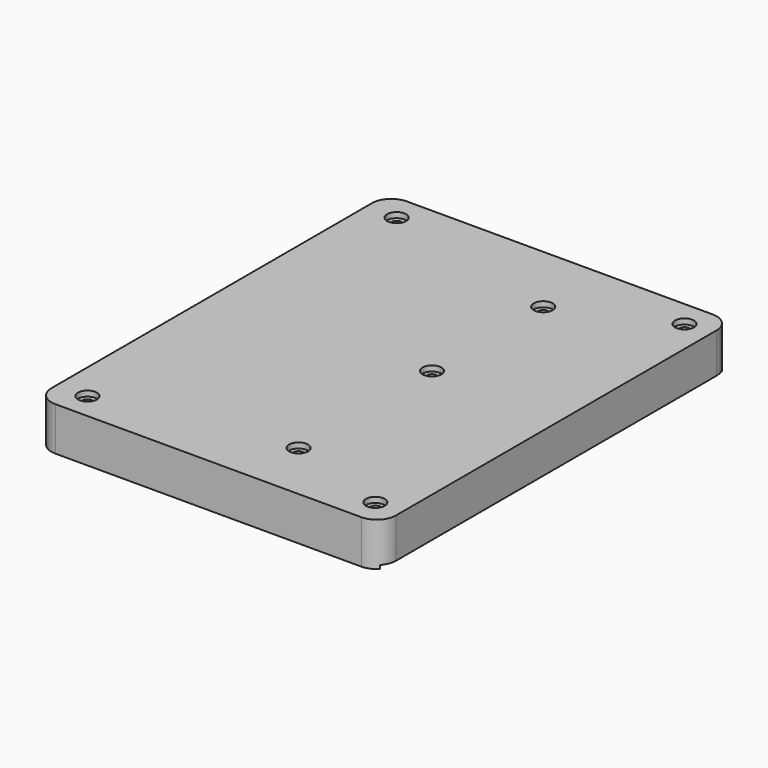
from build123d import *

# Parameters (mm, degrees)
F7_DEPTH        = 8.9
F9_DEPTH        = 0.8
F11_W           = 14.971
F11_H           = 45.903
F11_H_2         = 42.347
F13_DEPTH       = 7.1999999775
F14_DEPTH       = 5.9
F10_R           = 2.6
F16_R           = 3.5
F18_DEPTH       = 4.4
F19_SIZE        = 0.89999
F20_D           = 2.2
F20_CBORE_D     = 4.2
F20_CBORE_DEPTH = 1.2
F21_W           = 84.162
F21_H           = 95.25
F22_DEPTH       = 0.801


# Not quite as in the source:
# - a fillet or chamfer is up to 0.001 mm smaller than in the source, because OpenCascade refuses the exact size


with BuildPart() as f7:
    # F4 (on offset) → F7 (new body, through all)
    with BuildSketch(Plane.XY.offset(1.7)):
        with BuildLine():
            Line((84.612, 3), (84.612, 92.25))
            ThreePointArc((84.612, 92.25), (83.3525591591, 95.2905591591), (80.312, 96.55))
            Line((80.312, 96.55), (12.15, 96.55))
            ThreePointArc((12.15, 96.55), (9.1094408409, 95.2905591591), (7.85, 92.25))
            Line((7.85, 92.25), (7.85, 3))
            ThreePointArc((7.85, 3), (9.1094408409, -0.0405591591), (12.15, -1.3))
            Line((12.15, -1.3), (80.312, -1.3))
            ThreePointArc((80.312, -1.3), (83.3525591591, -0.0405591591), (84.612, 3))
        make_face()
    extrude(amount=F7_DEPTH)

    # F8 (on offset) → F9 (join)
    with BuildSketch(Plane.XY.offset(1.7)):
        with BuildLine():
            Line((84.612, 3), (84.612, 92.25))
            ThreePointArc((84.612, 92.25), (83.3525591591, 95.2905591591), (80.312, 96.55))
            Line((80.312, 96.55), (12.15, 96.55))
            ThreePointArc((12.15, 96.55), (9.1094408409, 95.2905591591), (7.85, 92.25))
            Line((7.85, 92.25), (7.85, 3))
            ThreePointArc((7.85, 3), (9.1094408409, -0.0405591591), (12.15, -1.3))
            Line((12.15, -1.3), (80.312, -1.3))
            ThreePointArc((80.312, -1.3), (83.3525591591, -0.0405591591), (84.612, 3))
        make_face()
        with BuildLine():
            ThreePointArc((80.312, 95.25), (82.4333203436, 94.3713203436), (83.312, 92.25))
            Line((83.312, 92.25), (83.312, 3))
            ThreePointArc((83.312, 3), (82.4333203436, 0.8786796564), (80.312, 0))
            Line((80.312, 0), (12.15, 0))
            ThreePointArc((12.15, 0), (10.0286796564, 0.8786796564), (9.15, 3))
            Line((9.15, 3), (9.15, 92.25))
            ThreePointArc((9.15, 92.25), (10.0286796564, 94.3713203436), (12.15, 95.25))
            Line((12.15, 95.25), (80.312, 95.25))
        make_face(mode=Mode.SUBTRACT)
    extrude(amount=-F9_DEPTH)

    # F11 (on offset) → F13 (cut, through all)
    with BuildSketch(Plane.XY.offset(1.7)):
        with BuildLine():
            Line((58.999, 0), (80.312, 0))
            ThreePointArc((80.312, 0), (82.4333203436, 0.8786796564), (83.312, 3))
            Line((83.312, 3), (83.312, 45.903))
            Line((83.312, 45.903), (58.999, 45.903))
            Line((58.999, 45.903), (58.999, 0))
        make_face()
        with Locations((44.5135, 22.9515)):
            Rectangle(F11_W, F11_H)
        with BuildLine():
            Line((9.15, 45.903), (9.15, 3))
            ThreePointArc((9.15, 3), (10.0286796564, 0.8786796564), (12.15, 0))
            Line((12.15, 0), (30.028, 0))
            Line((30.028, 0), (30.028, 45.903))
            Line((30.028, 45.903), (9.15, 45.903))
        make_face()
        with Locations((44.5135, 74.0765)):
            Rectangle(F11_W, F11_H_2)
        with BuildLine():
            Line((80.312, 95.25), (58.999, 95.25))
            Line((58.999, 95.25), (58.999, 52.903))
            Line((58.999, 52.903), (83.312, 52.903))
            Line((83.312, 52.903), (83.312, 92.25))
            ThreePointArc((83.312, 92.25), (82.4333203436, 94.3713203436), (80.312, 95.25))
        make_face()
        with BuildLine():
            ThreePointArc((12.15, 95.25), (10.0286796564, 94.3713203436), (9.15, 92.25))
            Line((9.15, 92.25), (9.15, 52.903))
            Line((9.15, 52.903), (30.028, 52.903))
            Line((30.028, 52.903), (30.028, 95.25))
            Line((30.028, 95.25), (12.15, 95.25))
        make_face()
    extrude(amount=F13_DEPTH, mode=Mode.SUBTRACT)

    # F8 (on offset) → F14 (cut, through all)
    with BuildSketch(Plane.XY.offset(1.7)):
        with BuildLine():
            Line((83.312, 3), (83.312, 92.25))
            ThreePointArc((83.312, 92.25), (82.4333203436, 94.3713203436), (80.312, 95.25))
            Line((80.312, 95.25), (12.15, 95.25))
            ThreePointArc((12.15, 95.25), (10.0286796564, 94.3713203436), (9.15, 92.25))
            Line((9.15, 92.25), (9.15, 3))
            ThreePointArc((9.15, 3), (10.0286796564, 0.8786796564), (12.15, 0))
            Line((12.15, 0), (80.312, 0))
            ThreePointArc((80.312, 0), (82.4333203436, 0.8786796564), (83.312, 3))
        make_face()
    extrude(amount=F14_DEPTH, mode=Mode.SUBTRACT)

    # F10 (on offset) → F15 (join, up to the next surface of F7)
    with BuildSketch(Plane.XY.offset(1.7)):
        with Locations((78.74, 90.678)):
            Circle(F10_R)
        with Locations((55.499, 80.3793147206)):
            Circle(F10_R)
        with Locations((14.608, 90.678)):
            Circle(F10_R)
        with Locations((55.499, 49.403)):
            Circle(F10_R)
        with Locations((14.608, 4.572)):
            Circle(F10_R)
        with Locations((55.499, 12.2474404052)):
            Circle(F10_R)
        with Locations((78.74, 4.572)):
            Circle(F10_R)
    extrude(until=Until.NEXT)

    # F16 (on offset) → F18 (join, through all)
    with BuildSketch(Plane.XY.offset(10.6)):
        with Locations((78.74, 4.572)):
            Circle(F16_R)
        with Locations((78.74, 90.678)):
            Circle(F16_R)
        with Locations((55.499, 80.3793147206)):
            Circle(F16_R)
        with Locations((55.499, 12.2474404052)):
            Circle(F16_R)
        with Locations((14.608, 90.678)):
            Circle(F16_R)
        with Locations((14.608, 4.572)):
            Circle(F16_R)
        with Locations((55.499, 49.403)):
            Circle(F16_R)
    extrude(amount=-F18_DEPTH)

    # F19 (size 0.9 in the source; OpenCascade refuses exactly that, so slightly less here)
    f19_edges = [f7.edges().sort_by_distance(p)[0] for p in [
        (75.24, 90.678, 6.2),
        (51.999, 80.379315, 6.2),
        (11.108, 90.678, 6.2),
        (51.999, 49.403, 6.2),
        (51.999, 12.24744, 6.2),
        (75.24, 4.572, 6.2),
        (11.108, 4.572, 6.2),
    ]]
    chamfer(f19_edges, length=F19_SIZE)

    # F20 (through all)
    with Locations(Plane.XY.offset(10.6)):
        with Locations((78.74, 90.678), (55.499, 80.3793147206), (55.499, 49.403), (14.608, 90.678), (55.499, 12.2474404052), (78.74, 4.572), (14.608, 4.572)):
            CounterBoreHole(F20_D / 2, F20_CBORE_D / 2, F20_CBORE_DEPTH)

    # F21 (on offset) → F22 (cut, through all)
    with BuildSketch(Plane.XY.offset(1.7)):
        with Locations((46.231, 47.625)):
            Rectangle(F21_W, F21_H)
    extrude(amount=-F22_DEPTH, mode=Mode.SUBTRACT)


solid = f7.part
